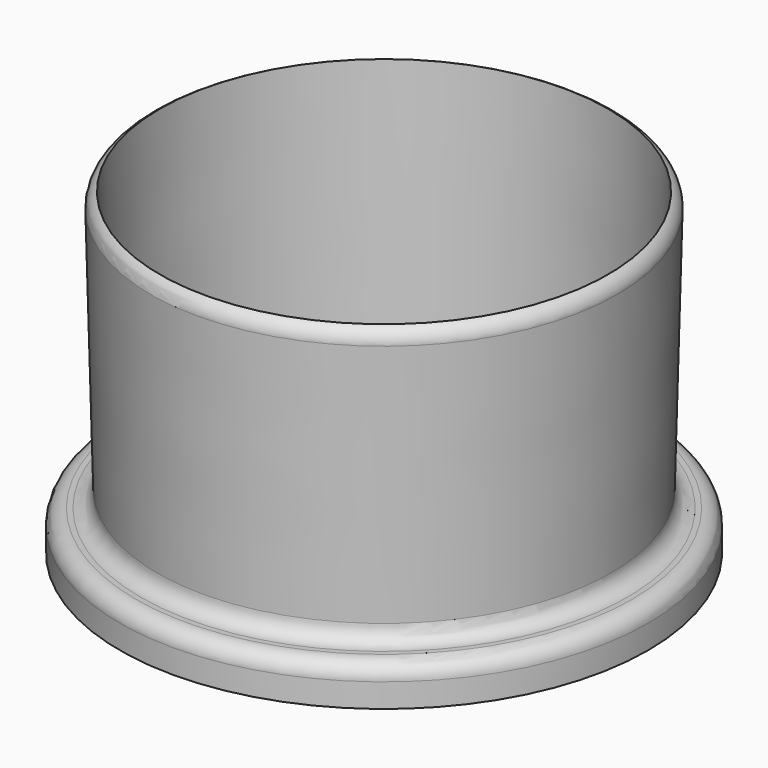
from build123d import *

# Parameters (mm, degrees)
F3_R     = 1.27
F4_DEPTH = 5.08


# Not quite as in the source:
# - a fillet or chamfer that OpenCascade refuses, or shapes differently, is made with other operations: its cross-section is extruded or revolved along the edge and cut away or added


with BuildPart() as f1:
    # F0 (on Front) → F1 (revolve)
    with BuildSketch(Plane.XZ):
        Polygon((-42.164, 0), (-34.544, 0), (-35.814, 50.8), (-37.314, 50.8), (-36.20275, 6.35), (-42.164, 6.35), align=None)
    revolve(axis=Axis((0, 0, 8.2894073013), (0, 0, -1)))

    # F2: fillet of radius 2.54 on 3 edges, made by hand

    # F2_s1 → F2_t2 (revolve)
    with BuildSketch(Plane.XZ):
        with BuildLine():
            ThreePointArc((-38.807043626, 6.35), (-36.9886872775, 7.1165344126), (-36.2678370041, 8.9534801655))
            Line((-36.2678370041, 8.9534801655), (-36.20275, 6.35))
            Line((-36.20275, 6.35), (-38.807043626, 6.35))
        make_face()
    revolve(axis=Axis((0, 0, 6.35), (0, 0, -1)))

    # F2_s3 → F2_t4 (revolve, cut)
    with BuildSketch(Plane.XZ):
        with BuildLine():
            ThreePointArc((-39.624, 6.35), (-41.4200512242, 5.6060512242), (-42.164, 3.81))
            Line((-42.164, 3.81), (-42.164, 6.35))
            Line((-42.164, 6.35), (-39.624, 6.35))
        make_face()
    revolve(axis=Axis((0, 0, 6.35), (0, 0, -1)), mode=Mode.SUBTRACT)

    # F2_s5 → F2_t6 (revolve, cut)
    with BuildSketch(Plane.XZ):
        with BuildLine():
            ThreePointArc((-37.2551532867, 48.4461314672), (-36.8821851711, 49.8358886527), (-35.814, 50.8))
            Line((-35.814, 50.8), (-37.314, 50.8))
            Line((-37.314, 50.8), (-37.2551532867, 48.4461314672))
        make_face()
    revolve(axis=Axis((0, 0, 50.8), (0, 0, -1)), mode=Mode.SUBTRACT)

    # F3 (on face) → F4 (cut)
    with BuildSketch(Plane(origin=(0, 0, 0), x_dir=(1, 0, 0), z_dir=(0, 0, -1))):
        with Locations((0, 38.1)):
            Circle(F3_R)
        with Locations((38.1, 0)):
            Circle(F3_R)
        with Locations((0, -38.1)):
            Circle(F3_R)
        with Locations((-38.1, 0)):
            Circle(F3_R)
    extrude(amount=-F4_DEPTH, mode=Mode.SUBTRACT)


solid = f1.part
